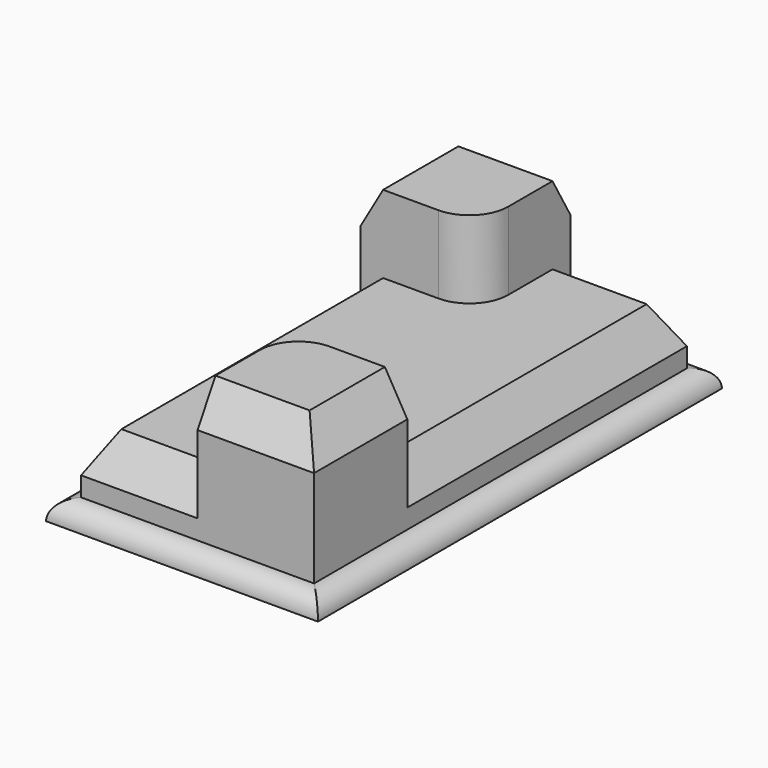
from build123d import *

# Parameters (mm, degrees)
F0_W       = 88.9
F0_H       = 165.1
F1_DEPTH   = 6.35
F2_DEPTH   = 25.4
F3_DEPTH   = 50.8
F4_SIZE2   = 12.7
F4_SIZE    = 7.3323484187
F4_2_SIZE2 = 12.7
F4_2_SIZE  = 7.3323484187
F4_3_SIZE2 = 12.7
F4_3_SIZE  = 7.3323484187
F5_R       = 6.34999


# Not quite as in the source:
# - a fillet or chamfer is up to 0.001 mm smaller than in the source, because OpenCascade refuses the exact size


with BuildPart() as f1:
    # F0 (on Top) → F1 (new body)
    with BuildSketch(Plane.XY):
        with Locations((-5.7064332783, -7.9358178854)):
            Rectangle(F0_W, F0_H)
        Polygon((-43.8064332783, 30.1641821146), (-43.8064332783, 68.2641821146), (-5.7064332783, 68.2641821146), (32.3935667217, 68.2641821146), (32.3935667217, -46.0358178854), (32.3935667217, -84.1358178854), (-5.7064332783, -84.1358178854), (-43.8064332783, -84.1358178854), align=None, mode=Mode.SUBTRACT)
    extrude(amount=F1_DEPTH)

    # F0 (on Top) → F2 (join)
    with BuildSketch(Plane.XY):
        with BuildLine():
            Line((-18.4064332783, 30.1641821146), (-43.8064332783, 30.1641821146))
            Line((-43.8064332783, 30.1641821146), (-43.8064332783, -84.1358178854))
            Line((-43.8064332783, -84.1358178854), (-5.7064332783, -84.1358178854))
            Line((-5.7064332783, -84.1358178854), (-5.7064332783, -58.7358178854))
            ThreePointArc((-5.7064332783, -58.7358178854), (-1.9866893994, -49.7555617643), (6.9935667217, -46.0358178854))
            Line((6.9935667217, -46.0358178854), (32.3935667217, -46.0358178854))
            Line((32.3935667217, -46.0358178854), (32.3935667217, 68.2641821146))
            Line((32.3935667217, 68.2641821146), (-5.7064332783, 68.2641821146))
            Line((-5.7064332783, 68.2641821146), (-5.7064332783, 42.8641821146))
            ThreePointArc((-5.7064332783, 42.8641821146), (-9.4261771573, 33.8839259935), (-18.4064332783, 30.1641821146))
        make_face()
    extrude(amount=F2_DEPTH)

    # F0 (on Top) → F3 (join)
    with BuildSketch(Plane.XY):
        with BuildLine():
            Line((-5.7064332783, 68.2641821146), (-43.8064332783, 68.2641821146))
            Line((-43.8064332783, 68.2641821146), (-43.8064332783, 30.1641821146))
            Line((-43.8064332783, 30.1641821146), (-18.4064332783, 30.1641821146))
            ThreePointArc((-18.4064332783, 30.1641821146), (-9.4261771573, 33.8839259935), (-5.7064332783, 42.8641821146))
            Line((-5.7064332783, 42.8641821146), (-5.7064332783, 68.2641821146))
        make_face()
        with BuildLine():
            Line((-5.7064332783, -58.7358178854), (-5.7064332783, -84.1358178854))
            Line((-5.7064332783, -84.1358178854), (32.3935667217, -84.1358178854))
            Line((32.3935667217, -84.1358178854), (32.3935667217, -46.0358178854))
            Line((32.3935667217, -46.0358178854), (6.9935667217, -46.0358178854))
            ThreePointArc((6.9935667217, -46.0358178854), (-1.9866893994, -49.7555617643), (-5.7064332783, -58.7358178854))
        make_face()
    extrude(amount=F3_DEPTH)

    # F4
    f4_edges = [f1.edges().sort_by_distance(p)[0] for p in [
        (-24.756433, -84.135818, 25.4),
        (32.393567, 11.114182, 25.4),
        (13.343567, 68.264182, 25.4),
        (-43.806433, -26.985818, 25.4),
    ]]
    f4_side = f1.faces().sort_by_distance((-5.706433, -7.935818, 25.4))[0]
    chamfer(f4_edges, length=F4_SIZE, length2=F4_SIZE2, reference=f4_side)

    # F4#2
    f4_2_edges = [f1.edges().sort_by_distance(p)[0] for p in [
        (-24.756433, 68.264182, 50.8),
        (-43.806433, 49.214182, 50.8),
    ]]
    f4_2_side = f1.faces().sort_by_distance((-25.152475, 49.610224, 50.8))[0]
    chamfer(f4_2_edges, length=F4_2_SIZE, length2=F4_2_SIZE2, reference=f4_2_side)

    # F4#3
    f4_3_edges = [f1.edges().sort_by_distance(p)[0] for p in [
        (13.343567, -84.135818, 50.8),
        (32.393567, -65.085818, 50.8),
    ]]
    f4_3_side = f1.faces().sort_by_distance((13.739609, -65.48186, 50.8))[0]
    chamfer(f4_3_edges, length=F4_3_SIZE, length2=F4_3_SIZE2, reference=f4_3_side)

    # F5 (radius 6.35 in the source; OpenCascade refuses exactly that, so slightly less here)
    f5_edges = [f1.edges().sort_by_distance(p)[0] for p in [
        (38.743567, -7.935818, 6.35),
        (-5.706433, 74.614182, 6.35),
        (-50.156433, -7.935818, 6.35),
        (-5.706433, -90.485818, 6.35),
    ]]
    fillet(f5_edges, radius=F5_R)


solid = f1.part
